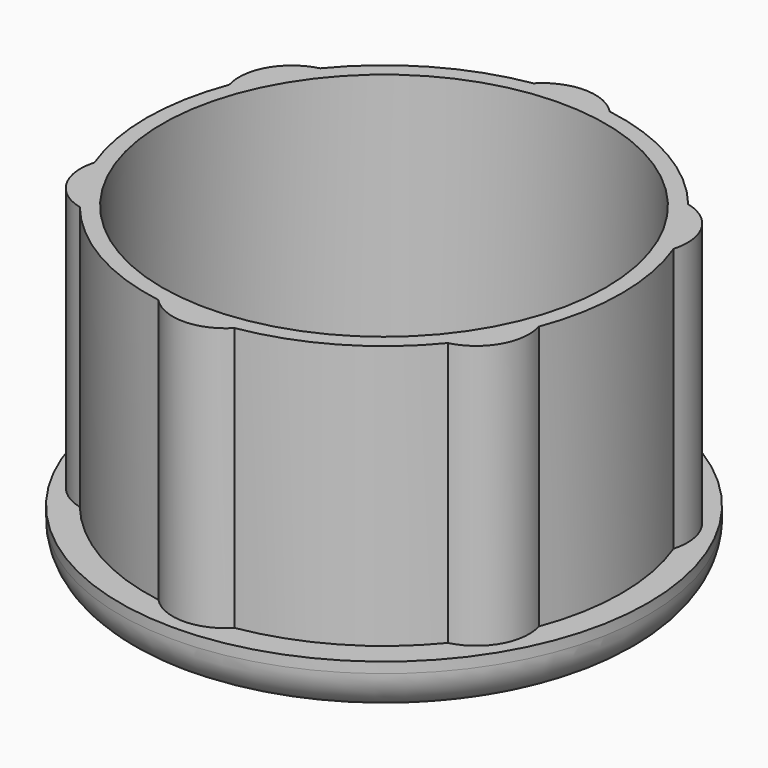
from build123d import *

# Parameters (mm, degrees)
F0_R            = 10
F1_DEPTH        = 2
F2_R            = 1.6
F4_R            = 9
F4_R_2          = 8.4
F5_DEPTH        = 10
F7_DEPTH        = 10
F7_COPIES_COUNT = 6


# Not quite as in the source:
# - a pattern or mirror of a feature is missing from the dataset's text; its kind, count and spacing are read off the source's solid


with BuildPart() as f1:
    # F0 (on Top) → F1 (new body)
    with BuildSketch(Plane.XY):
        Circle(F0_R)
    extrude(amount=F1_DEPTH)

    # F2
    f2_edges = [f1.edges().sort_by_distance(p)[0] for p in [
        (-10, 0, 0),
    ]]
    fillet(f2_edges, radius=F2_R)

    # F4 (on face) → F5 (join)
    with BuildSketch(Plane.XY.offset(2)):
        Circle(F4_R)
        Circle(F4_R_2, mode=Mode.SUBTRACT)
    extrude(amount=F5_DEPTH)

    # F6 (on face) → F7 (join, through all)
    with BuildSketch(Plane.XY.offset(2)):
        with BuildLine():
            ThreePointArc((-1.4444337606, 8.8833333333), (0, 9), (1.4444337606, 8.8833333333))
            ThreePointArc((1.4444337606, 8.8833333333), (0, 9.5), (-1.4444337606, 8.8833333333))
        make_face()
    f7 = extrude(amount=F7_DEPTH)

    # F7_copies: F7 ×6 about axis
    f7_copies_axis = Axis((0, 0, 0), (0, 0, 1))
    for i in range(1, F7_COPIES_COUNT):
        add(f7.rotate(f7_copies_axis, i * 360 / F7_COPIES_COUNT))


solid = f1.part
